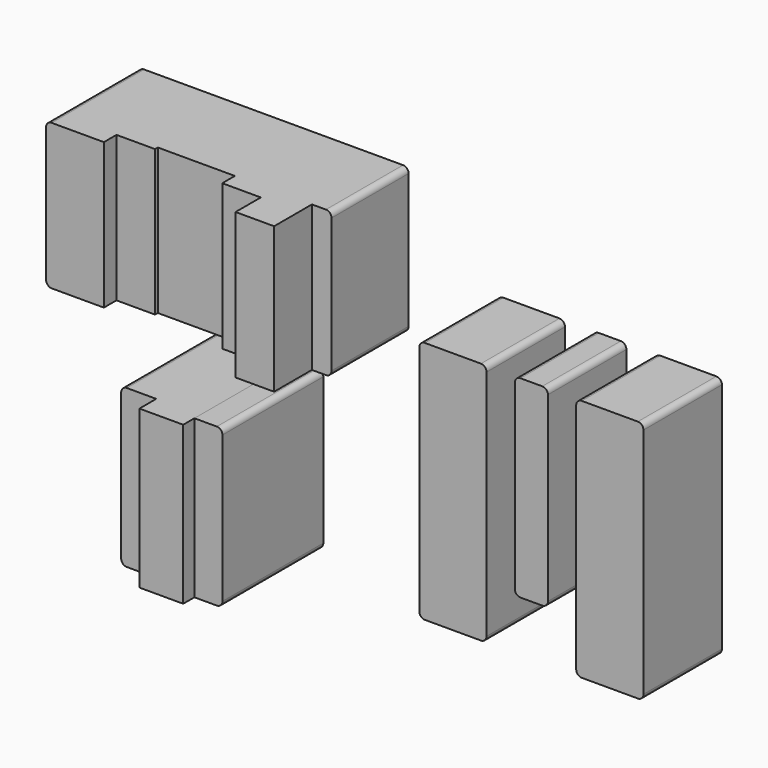
from build123d import *

# Parameters (mm, degrees)
F0_W      = 60.96
F0_H      = 220.98
F1_DEPTH  = 88.9
F0_W_2    = 29.972
F0_H_2    = 175.006
F2_R      = 5.08
F2_2_R    = 5.08
F2_3_R    = 5.08
F3_R      = 5.08
F0_W_3    = 52.3875
F0_H_3    = 132.08
F4_DEPTH  = 104.775
F0_W_4    = 34.925
F5_DEPTH  = 90.5002
F0_W_5    = 69.85
F6_DEPTH  = 87.3252
F7_DEPTH  = 101.6
F8_DEPTH  = 130.175
F0_W_6    = 17.78
F9_DEPTH  = 87.3252
F0_W_7    = 31.75
F0_H_4    = 142.875
F10_DEPTH = 107.95
F0_W_8    = 39.6875
F11_DEPTH = 127
F0_W_9    = 25.4
F12_DEPTH = 114.3
F13_R     = 5.08
F13_2_R   = 5.08
F13_3_R   = 5.08


with BuildPart() as f1:
    # F0 (on Front) → F1 (new body)
    with BuildSketch(Plane.XZ):
        with Locations((432.2953, -250.19)):
            Rectangle(F0_W, F0_H)
    extrude(amount=F1_DEPTH)

    # F2
    f2_edges = [f1.edges().sort_by_distance(p)[0] for p in [
        (462.7753, -44.45, -139.7),
        (401.8153, -44.45, -139.7),
        (401.8153, -44.45, -360.68),
        (462.7753, -44.45, -360.68),
    ]]
    fillet(f2_edges, radius=F2_R)


with BuildPart() as f1b:
    # F0 (on Front) → F1, piece 2 (new body)
    with BuildSketch(Plane.XZ):
        with Locations((574.5353, -250.19)):
            Rectangle(F0_W, F0_H)
    extrude(amount=F1_DEPTH)

    # F2#2
    f2_2_edges = [f1b.edges().sort_by_distance(p)[0] for p in [
        (605.0153, -44.45, -139.7),
        (544.0553, -44.45, -139.7),
        (544.0553, -44.45, -360.68),
        (605.0153, -44.45, -360.68),
    ]]
    fillet(f2_2_edges, radius=F2_2_R)


with BuildPart() as f1c:
    # F0 (on Front) → F1, piece 3 (new body)
    with BuildSketch(Plane.XZ):
        with Locations((503.4153, -227.203)):
            Rectangle(F0_W_2, F0_H_2)
    extrude(amount=F1_DEPTH)

    # F2#3
    f2_3_edges = [f1c.edges().sort_by_distance(p)[0] for p in [
        (518.4013, -44.45, -139.7),
        (488.4293, -44.45, -314.706),
        (518.4013, -44.45, -314.706),
    ]]
    fillet(f2_3_edges, radius=F2_3_R)

    # F3
    f3_edges = [f1c.edges().sort_by_distance(p)[0] for p in [
        (488.4293, -44.45, -139.7),
    ]]
    fillet(f3_edges, radius=F3_R)


with BuildPart() as f4:
    # F0 (on Front) → F4 (new body)
    with BuildSketch(Plane.XZ):
        with Locations((102.39375, -129.54)):
            Rectangle(F0_W_3, F0_H_3)
    extrude(amount=F4_DEPTH)

    # F0 (on Front) → F5 (join)
    with BuildSketch(Plane.XZ):
        with Locations((146.05, -129.54)):
            Rectangle(F0_W_4, F0_H_3)
    extrude(amount=F5_DEPTH)

    # F0 (on Front) → F6 (join)
    with BuildSketch(Plane.XZ):
        with Locations((198.4375, -129.54)):
            Rectangle(F0_W_5, F0_H_3)
    extrude(amount=F6_DEPTH)

    # F0 (on Front) → F7 (join)
    with BuildSketch(Plane.XZ):
        with Locations((250.825, -129.54)):
            Rectangle(F0_W_4, F0_H_3)
    extrude(amount=F7_DEPTH)

    # F0 (on Front) → F8 (join)
    with BuildSketch(Plane.XZ):
        with Locations((285.75, -129.54)):
            Rectangle(F0_W_4, F0_H_3)
    extrude(amount=F8_DEPTH)

    # F0 (on Front) → F9 (join)
    with BuildSketch(Plane.XZ):
        with Locations((312.1025, -129.54)):
            Rectangle(F0_W_6, F0_H_3)
    extrude(amount=F9_DEPTH)

    # F13
    f13_edges = [f4.edges().sort_by_distance(p)[0] for p in [
        (320.9925, -43.6626, -63.5),
        (76.2, -52.3875, -63.5),
        (320.9925, -43.6626, -195.58),
        (76.2, -52.3875, -195.58),
    ]]
    fillet(f13_edges, radius=F13_R)


with BuildPart() as f10:
    # F0 (on Front) → F10 (new body)
    with BuildSketch(Plane.XZ):
        with Locations((162.7124, -322.2625)):
            Rectangle(F0_W_7, F0_H_4)
    extrude(amount=F10_DEPTH)

    # F0 (on Front) → F11 (join)
    with BuildSketch(Plane.XZ):
        with Locations((198.43115, -322.2625)):
            Rectangle(F0_W_8, F0_H_4)
    extrude(amount=F11_DEPTH)

    # F13#2
    f13_2_edges = [f10.edges().sort_by_distance(p)[0] for p in [
        (146.8374, -53.975, -250.825),
        (146.8374, -53.975, -393.7),
    ]]
    fillet(f13_2_edges, radius=F13_2_R)


with BuildPart() as f12:
    # F0 (on Front) → F12 (new body)
    with BuildSketch(Plane.XZ):
        with Locations((230.9749, -322.2625)):
            Rectangle(F0_W_9, F0_H_4)
    extrude(amount=F12_DEPTH)

    # F13#3
    f13_3_edges = [f12.edges().sort_by_distance(p)[0] for p in [
        (243.6749, -57.15, -250.825),
        (243.6749, -57.15, -393.7),
    ]]
    fillet(f13_3_edges, radius=F13_3_R)


solid = Compound([f1.part, f1b.part, f1c.part, f4.part, f10.part, f12.part])
